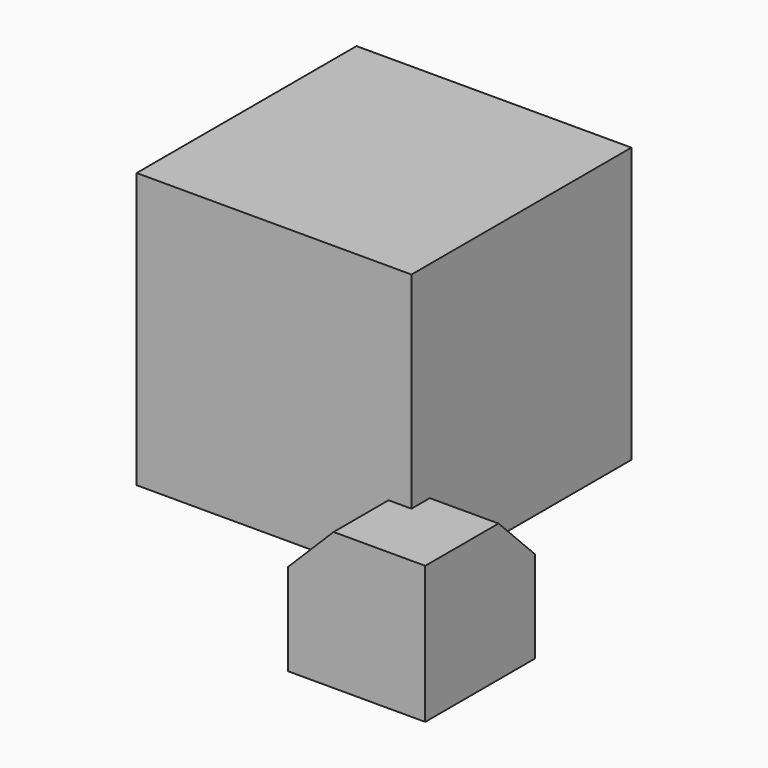
from build123d import *

# Parameters (mm, degrees)
F0_W     = 19.05
F0_H     = 19.05
F1_DEPTH = 19.05
F4_DEPTH = 9.525
F6_DEPTH = 13.8938
F8_DEPTH = 12.192


# Not quite as in the source:
# - a feature names something its author has since deleted; it is built from what else it names


with BuildPart() as f1:
    # F0 (on Front) → F1 (new body)
    with BuildSketch(Plane.XZ):
        with Locations((9.525, 9.525)):
            Rectangle(F0_W, F0_H)
    extrude(amount=-F1_DEPTH)


with BuildPart() as f4:
    # F3 (on offset) → F4 (new body)
    with BuildSketch(Plane.XZ.offset(-4.7625)):
        Polygon((23.8125, 4.7625), (17.4625, 4.7625), (14.2875, 1.5875), (14.2875, -4.7625), (23.8125, -4.7625), align=None)
    extrude(amount=F4_DEPTH)

    # F5 (on face) → F6 (cut)
    with BuildSketch(Plane.YZ.offset(23.8125)):
        Polygon((4.7625, 4.7625), (1.5875, 4.7625), (4.7625, 1.5875), align=None)
    extrude(amount=-F6_DEPTH, mode=Mode.SUBTRACT)

    # F7 (on face) → F8 (cut)
    with BuildSketch(Plane(origin=(0, 0, -4.7625), x_dir=(1, 0, 0), z_dir=(0, 0, -1))):
        Polygon((14.2875, -1.5875), (14.2875, -4.7625), (17.4625, -4.7625), align=None)
    extrude(amount=-F8_DEPTH, mode=Mode.SUBTRACT)


solid = Compound([f1.part, f4.part])
